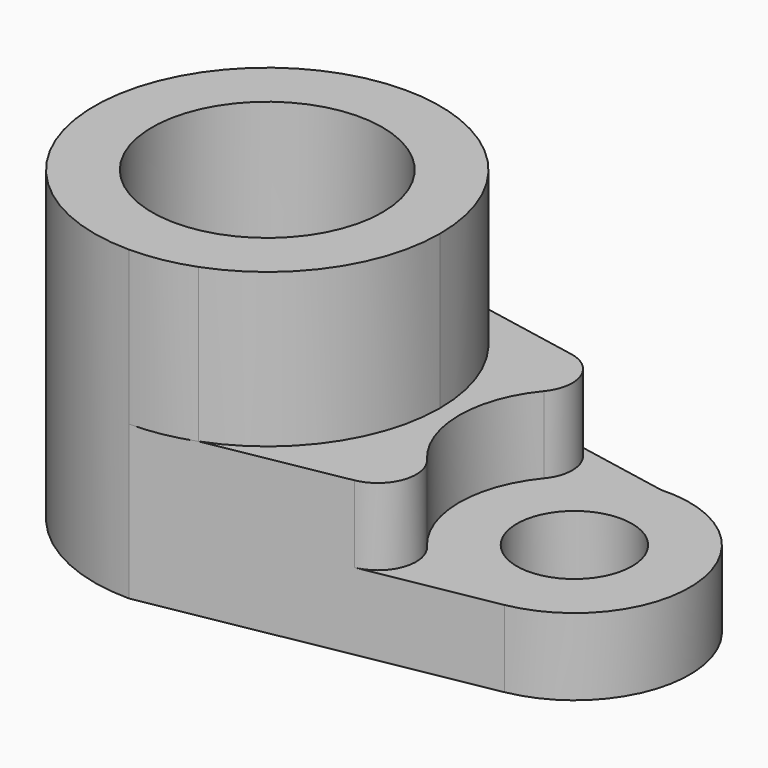
from build123d import *

# Parameters (mm, degrees)
F0_R        = 19.05
F0_R_2      = 9.525
F1_DEPTH    = 25.4
F2_DEPTH    = 25.4
F3_DEPTH    = 12.7
F4_T1_DEPTH = 57.2245179891
F4_T3_DEPTH = 67.6926131403


# Not quite as in the source:
# - a fillet or chamfer that OpenCascade refuses, or shapes differently, is made with other operations: its cross-section is extruded or revolved along the edge and cut away or added


with BuildPart() as f1:
    # F0 (on Top) → F1 (new body)
    with BuildSketch(Plane.XY):
        with BuildLine():
            Line((10.5539222721, 26.5545730464), (0, 28.575))
            ThreePointArc((0, 28.575), (-28.575, 0), (0, -28.575))
            Line((0, -28.575), (10.035773719, -26.7546981082))
            ThreePointArc((10.035773719, -26.7546981082), (23.4872610048, -16.2751096921), (28.575, 0))
            ThreePointArc((28.575, 0), (23.644332872, 16.046063319), (10.5539222721, 26.5545730464))
        make_face()
        Circle(F0_R, mode=Mode.SUBTRACT)
        with BuildLine():
            Line((49.8728171001, 19.0274231537), (10.5539222721, 26.5545730464))
            ThreePointArc((10.5539222721, 26.5545730464), (23.644332872, 16.046063319), (28.575, 0))
            ThreePointArc((28.575, 0), (23.4872610048, -16.2751096921), (10.035773719, -26.7546981082))
            Line((10.035773719, -26.7546981082), (54.1998407335, -18.7441613039))
            ThreePointArc((54.1998407335, -18.7441613039), (31.8737838621, -2.1681426844), (49.8728171001, 19.0274231537))
        make_face()
        with BuildLine():
            ThreePointArc((69.85, 0), (63.9384867043, 13.7942983555), (49.8728171001, 19.0274231537))
            ThreePointArc((49.8728171001, 19.0274231537), (31.8737838621, -2.1681426844), (54.1998407335, -18.7441613039))
            ThreePointArc((54.1998407335, -18.7441613039), (65.4230890371, -12.2093311452), (69.85, 0))
        make_face()
        with Locations((50.8, 0)):
            Circle(F0_R_2, mode=Mode.SUBTRACT)
    extrude(amount=-F1_DEPTH)

    # F0 (on Top) → F2 (join)
    with BuildSketch(Plane.XY):
        with BuildLine():
            Line((10.5539222721, 26.5545730464), (0, 28.575))
            ThreePointArc((0, 28.575), (-28.575, 0), (0, -28.575))
            Line((0, -28.575), (10.035773719, -26.7546981082))
            ThreePointArc((10.035773719, -26.7546981082), (23.4872610048, -16.2751096921), (28.575, 0))
            ThreePointArc((28.575, 0), (23.644332872, 16.046063319), (10.5539222721, 26.5545730464))
        make_face()
        Circle(F0_R, mode=Mode.SUBTRACT)
        with BuildLine():
            Line((10.035773719, -26.7546981082), (0, -28.575))
            ThreePointArc((0, -28.575), (5.0997611002, -28.1162419559), (10.035773719, -26.7546981082))
        make_face()
        with BuildLine():
            ThreePointArc((10.5539222721, 26.5545730464), (5.3727879262, 28.0653482947), (0, 28.575))
            Line((0, 28.575), (10.5539222721, 26.5545730464))
        make_face()
    extrude(amount=F2_DEPTH)

    # F0 (on Top) → F3 (cut)
    with BuildSketch(Plane.XY):
        with BuildLine():
            ThreePointArc((69.85, 0), (63.9384867043, 13.7942983555), (49.8728171001, 19.0274231537))
            ThreePointArc((49.8728171001, 19.0274231537), (31.8737838621, -2.1681426844), (54.1998407335, -18.7441613039))
            ThreePointArc((54.1998407335, -18.7441613039), (65.4230890371, -12.2093311452), (69.85, 0))
        make_face()
        with Locations((50.8, 0)):
            Circle(F0_R_2, mode=Mode.SUBTRACT)
    extrude(amount=-F3_DEPTH, mode=Mode.SUBTRACT)

    # F4: fillet of radius 6.35 on 3 edges, made by hand

    # F4_s2 → F4_t1 (cut)
    with BuildSketch(Plane.XY.offset(-12.7)):
        with BuildLine():
            ThreePointArc((32.3806581498, 22.376095667), (37.1591875386, 18.2961908719), (36.0900289579, 12.1045137012))
            ThreePointArc((36.0900289579, 12.1045137012), (42.2494552996, 17.0232395662), (49.8728171001, 19.0274231537))
            Line((49.8728171001, 19.0274231537), (32.3806581498, 22.376095667))
        make_face()
    extrude(amount=F4_T1_DEPTH, mode=Mode.SUBTRACT)

    # F4_s4 → F4_t3 (cut)
    with BuildSketch(Plane.XY.offset(-12.7)):
        with BuildLine():
            ThreePointArc((32.5559475844, -22.6699592292), (37.4002807494, -18.5644828639), (36.2670005049, -12.3164290959))
            ThreePointArc((36.2670005049, -12.3164290959), (44.372267792, -17.9328402285), (54.1998407335, -18.7441613039))
            Line((54.1998407335, -18.7441613039), (32.5559475844, -22.6699592292))
        make_face()
    extrude(amount=F4_T3_DEPTH, mode=Mode.SUBTRACT)


solid = f1.part
